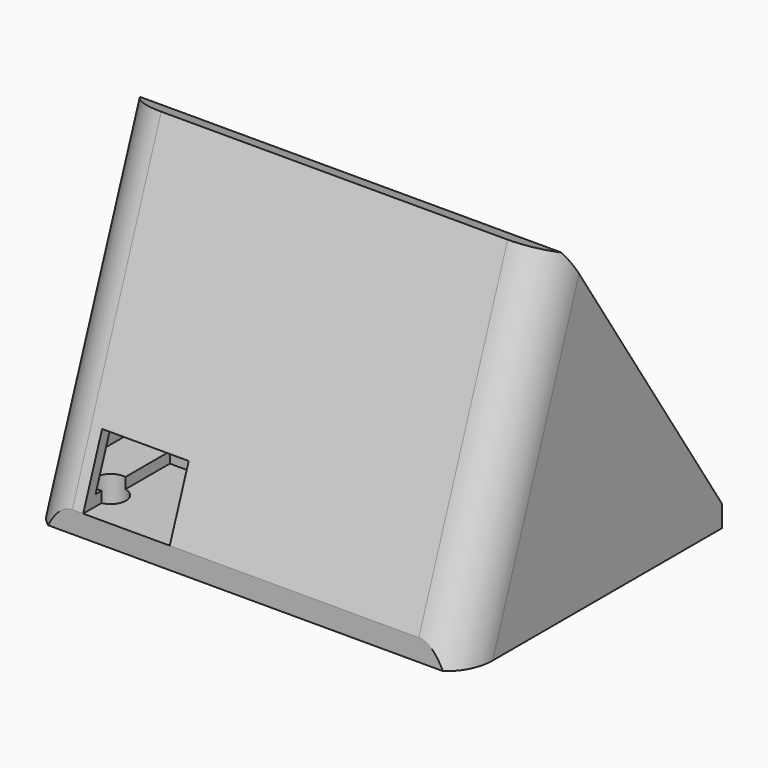
from build123d import *

# Parameters (mm, degrees)
F1_DEPTH = 40
F2_T     = -1
F0_W     = 30
F0_H     = 2
F3_DEPTH = 40
F4_W     = 8
F4_H     = 6
F5_DEPTH = 10
F6_R     = 1.4
F7_DEPTH = 3
F8_R     = 4


with BuildPart() as f1:
    # F0 (on Right) → F1 (new body)
    with BuildSketch(Plane.YZ):
        Polygon((10.2606042998, 28.1907786236), (0, 0), (30, 0), (12.1399895413, 27.5067383369), align=None)
    extrude(amount=F1_DEPTH)

    # F2
    f2_openings = [f1.faces().sort_by_distance(p)[0] for p in [
        (20, 21.069995, 13.753369),
    ]]
    offset(amount=F2_T, openings=f2_openings, kind=Kind.INTERSECTION)

    # F0 (on Right) → F3 (join)
    with BuildSketch(Plane.YZ):
        with Locations((15, -1)):
            Rectangle(F0_W, F0_H)
    extrude(amount=F3_DEPTH)

    # F4 (on Front) → F5 (cut)
    with BuildSketch(Plane.XZ):
        with Locations((9, 3)):
            Rectangle(F4_W, F4_H)
    extrude(amount=-F5_DEPTH, mode=Mode.SUBTRACT)

    # F6 (on face) → F7 (cut)
    with BuildSketch(Plane(origin=(0, 0, -2), x_dir=(1, 0, 0), z_dir=(0, 0, -1))):
        with Locations((4.75, -3.5)):
            Circle(F6_R)
        with Locations((35.25, -3.5)):
            Circle(F6_R)
    extrude(amount=-F7_DEPTH, mode=Mode.SUBTRACT)

    # F8
    f8_edges = [f1.edges().sort_by_distance(p)[0] for p in [
        (1, 6.143212, 13.954533),
        (39, 6.143212, 13.954533),
        (0, 5.130302, 14.095389),
        (40, 5.130302, 14.095389),
    ]]
    fillet(f8_edges, radius=F8_R)


solid = f1.part
